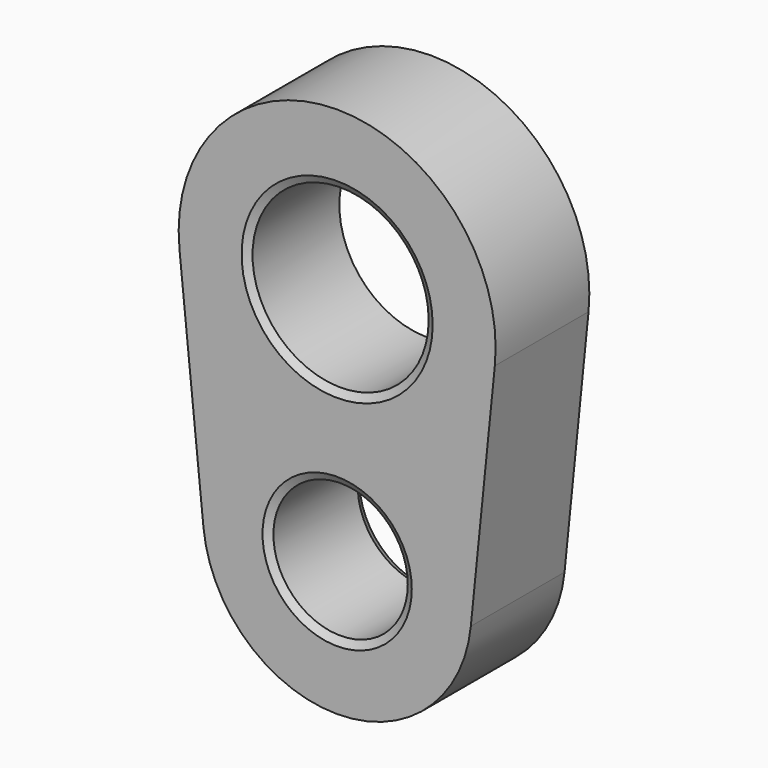
from build123d import *

# Parameters (mm, degrees)
F0_R        = 1.9812
F0_R_2      = 2.59715
F1_DEPTH    = 3.4544
F2_C1_SIZE2 = 0.127
F2_C1_SIZE  = 0.2199704526
F2_C2_SIZE2 = 0.2199704526
F2_C2_SIZE  = 0.127
F2_C3_SIZE2 = 0.127
F2_C3_SIZE  = 0.2199704526
F2_C4_SIZE2 = 0.2199704526
F2_C4_SIZE  = 0.127


with BuildPart() as f1:
    # F0 (on Front) → F1 (new body)
    with BuildSketch(Plane.XZ):
        with BuildLine():
            Line((-4.6498341341, -0.4707223022), (-3.9422506789, -7.4602906475))
            ThreePointArc((-3.9422506789, -7.4602906475), (0, -11.0236), (3.9422506789, -7.4602906475))
            Line((3.9422506789, -7.4602906475), (4.6498341341, -0.4707223022))
            ThreePointArc((4.6498341341, -0.4707223022), (0, 4.6736), (-4.6498341341, -0.4707223022))
        make_face()
        with Locations((0, -7.0612)):
            Circle(F0_R, mode=Mode.SUBTRACT)
        Circle(F0_R_2, mode=Mode.SUBTRACT)
    extrude(amount=F1_DEPTH)

    # F2: chamfer of 0.127 x 0.2199704526 on 4 edges, made by hand

    # F2_c1
    f2_c1_edges = [f1.edges().sort_by_distance(p)[0] for p in [
        (-1.9812, 0, -7.0612),
    ]]
    f2_c1_side = f1.faces().sort_by_distance((-1.9812, -0.00254, -7.0612))[0]
    chamfer(f2_c1_edges, length=F2_C1_SIZE, length2=F2_C1_SIZE2, reference=f2_c1_side)

    # F2_c2
    f2_c2_edges = [f1.edges().sort_by_distance(p)[0] for p in [
        (-1.9812, -3.4544, -7.0612),
    ]]
    f2_c2_side = f1.faces().sort_by_distance((-1.9812, -3.45186, -7.0612))[0]
    chamfer(f2_c2_edges, length=F2_C2_SIZE, length2=F2_C2_SIZE2, reference=f2_c2_side)

    # F2_c3
    f2_c3_edges = [f1.edges().sort_by_distance(p)[0] for p in [
        (-2.59715, 0, 0),
    ]]
    f2_c3_side = f1.faces().sort_by_distance((-2.59969, 0, 0))[0]
    chamfer(f2_c3_edges, length=F2_C3_SIZE, length2=F2_C3_SIZE2, reference=f2_c3_side)

    # F2_c4
    f2_c4_edges = [f1.edges().sort_by_distance(p)[0] for p in [
        (-2.59715, -3.4544, 0),
    ]]
    f2_c4_side = f1.faces().sort_by_distance((-2.59715, -3.45186, 0))[0]
    chamfer(f2_c4_edges, length=F2_C4_SIZE, length2=F2_C4_SIZE2, reference=f2_c4_side)


solid = f1.part
